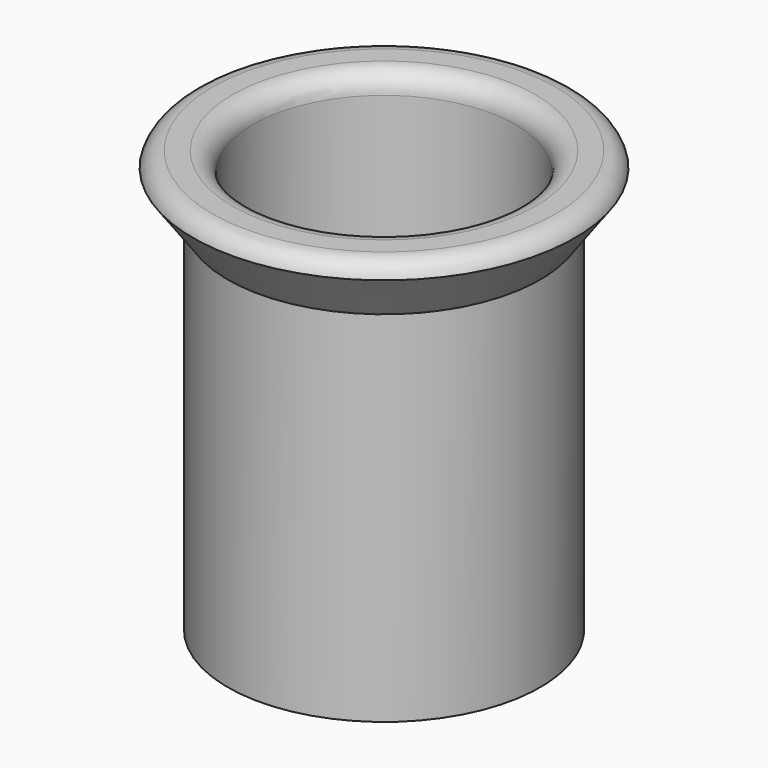
from build123d import *

# Parameters (mm, degrees)
F4_D = 25.4


# Not quite as in the source:
# - a fillet or chamfer that OpenCascade refuses, or shapes differently, is made with other operations: its cross-section is extruded or revolved along the edge and cut away or added


with BuildPart() as f1:
    # F0 (on Front) → F1 (revolve)
    with BuildSketch(Plane.XZ):
        Polygon((-33.655, 107.95), (-40.005, 107.95), (-48.8566160202, 107.95), (-48.8566160202, 104.1120141745), (-40.005, 91.8462350965), (-40.005, 0), (0, 0), (0, 6.35), (-33.655, 6.35), align=None)
    revolve(axis=Axis((0, 0, 3.175), (0, 0, -1)))

    # F2: fillet of radius 5.08 on 2 edges, made by hand

    # F2_s1 → F2_t2 (revolve, cut)
    with BuildSketch(Plane.XZ):
        with BuildLine():
            ThreePointArc((-33.655, 102.87), (-35.1428975516, 106.4621024484), (-38.735, 107.95))
            Line((-38.735, 107.95), (-33.655, 107.95))
            Line((-33.655, 107.95), (-33.655, 102.87))
        make_face()
    revolve(axis=Axis((0, 0, 107.95), (0, 0, -1)), mode=Mode.SUBTRACT)

    # F2_s3 → F2_t4 (revolve, cut)
    with BuildSketch(Plane.XZ):
        with BuildLine():
            ThreePointArc((-43.9307860606, 107.95), (-47.0530422956, 106.8772329609), (-48.8566160202, 104.1120141745))
            Line((-48.8566160202, 104.1120141745), (-48.8566160202, 107.95))
            Line((-48.8566160202, 107.95), (-43.9307860606, 107.95))
        make_face()
    revolve(axis=Axis((0, 0, 107.95), (0, 0, -1)), mode=Mode.SUBTRACT)

    # F4 (through all)
    with Locations(Plane(origin=(0, 0, 0), x_dir=(1, 0, 0), z_dir=(0, 0, -1))):
        with Locations((0, 0)):
            Hole(F4_D / 2)


solid = f1.part
